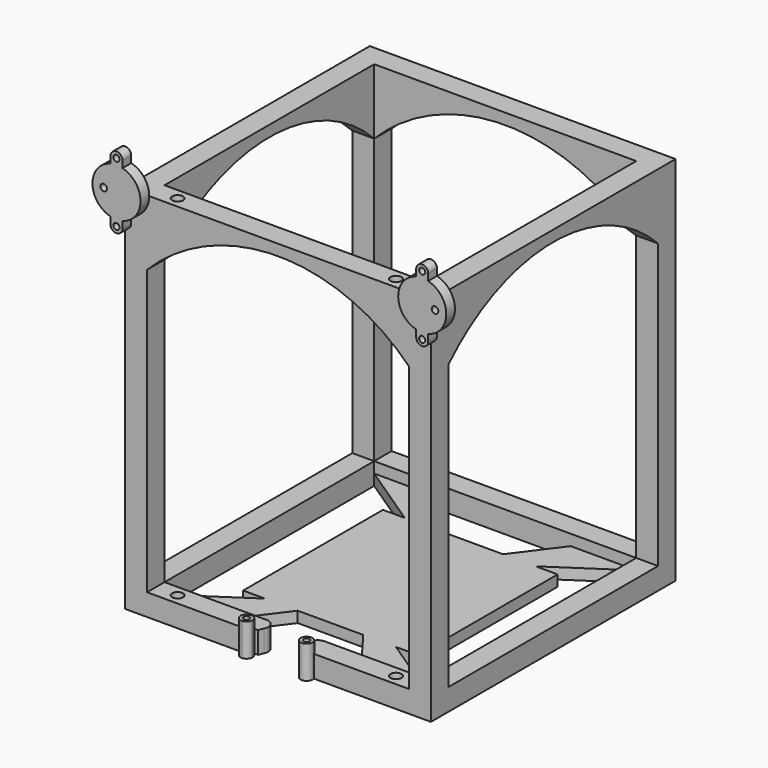
from build123d import *

# Parameters (mm, degrees)
F0_W      = 101.6
F0_H      = 101.6
F1_DEPTH  = 6.35
F2_W      = 12.7
F2_H      = 12.7
F3_DEPTH  = 88.9
F5_W      = 12.7
F5_H      = 12.7
F6_DEPTH  = 76.2
F9_W      = 38.1
F9_H      = 6.35
F8_W      = 19.05
F8_H      = 6.35
F14_W     = 12.7
F14_H     = 12.7
F15_DEPTH = 203.2
F17_DEPTH = 12.7
F20_DEPTH = 12.7
F22_R     = 3.175
F23_DEPTH = 209.55
F24_R     = 1.905
F24_R_2   = 1.778
F25_DEPTH = 19.05
F27_DEPTH = 25.4
F28_R     = 5.08
F29_R     = 1.778
F29_R_2   = 1.905
F30_DEPTH = 6.35


# Not quite as in the source:
# - a feature of the source that left no trace in its solid (it failed there, or was rolled back) is left out


with BuildPart() as f1:
    # F0 (on Top) → F1 (new body)
    with BuildSketch(Plane.XY):
        Rectangle(F0_W, F0_H)
    extrude(amount=-F1_DEPTH)



with BuildPart() as f3:
    # F2 (on Right) → F3 (new body, symmetric)
    with BuildSketch(Plane.YZ):
        with Locations((-82.55, 0)):
            Rectangle(F2_W, F2_H)
    extrude(amount=F3_DEPTH, both=True)


with BuildPart() as f4_1:
    # F4: instance of F3
    add(f3.part.mirror(Plane.XZ))


with BuildPart() as f3_1:
    add(f3.part)

    add(f4_1.part)  # F6 merges F4_1
    # F5 (on Front) → F6 (join, symmetric)
    with BuildSketch(Plane.XZ):
        with Locations((82.55, 0)):
            Rectangle(F5_W, F5_H)
    extrude(amount=F6_DEPTH, both=True)


with BuildPart() as f7_1:
    # F7: instance of F3
    add(f3_1.part.mirror(Plane.YZ))


with BuildPart() as f1_1:
    add(f1.part)

    add(f3_1.part)  # F10 merges F3

    add(f7_1.part)  # F10 merges F7_1
    # F9 (on face) → F10 section 0
    with BuildSketch(Plane(origin=(0, -76.2, 0), x_dir=(-1, 0, 0), z_dir=(0, 1, 0))):
        with Locations((57.15, -3.175)):
            Rectangle(F9_W, F9_H)
    # F8 (on face) → F10 section 1
    with BuildSketch(Plane.XZ.offset(50.8)):
        with Locations((-28.575, -3.175)):
            Rectangle(F8_W, F8_H)
    loft()


with BuildPart() as f11_1:
    # F11: instance of F1
    add(f1_1.part.mirror(Plane.YZ))


with BuildPart() as f12_1:
    # F12: instance of F11_1
    add(f11_1.part.mirror(Plane.XZ))


with BuildPart() as f12_2:
    # F12: instance of F1
    add(f1_1.part.mirror(Plane.XZ))


with BuildPart() as f1_2:
    add(f1_1.part)

    # F13: union F12_2, F11_1, F12_1
    add(f12_2.part)
    add(f11_1.part)
    add(f12_1.part)

    # F14 (on face) → F15 (join)
    with BuildSketch(Plane.XY.offset(6.35)):
        with Locations((-82.55, 82.55)):
            Rectangle(F14_W, F14_H)
        with Locations((82.55, 82.55)):
            Rectangle(F14_W, F14_H)
        with Locations((82.55, -82.55)):
            Rectangle(F14_W, F14_H)
        with Locations((-82.55, -82.55)):
            Rectangle(F14_W, F14_H)
    extrude(amount=F15_DEPTH)

    # F16 (on face) → F17 (join)
    with BuildSketch(Plane(origin=(-88.9, 0, 0), x_dir=(0, -1, 0), z_dir=(-1, 0, 0))):
        with BuildLine():
            ThreePointArc((-76.2, 171.45), (0, 203.2), (76.2, 171.45))
            Line((76.2, 171.45), (76.2, 209.55))
            Line((76.2, 209.55), (-76.2, 209.55))
            Line((-76.2, 209.55), (-76.2, 171.45))
        make_face()
    extrude(amount=-F17_DEPTH)

    # F18: F1 across plane


with BuildPart() as f1_3:
    add(f1_2.part)
    add(f1_2.part.mirror(Plane.YZ))

    # F19 (on face) → F20 (join)
    with BuildSketch(Plane(origin=(0, 88.9, 0), x_dir=(-1, 0, 0), z_dir=(0, 1, 0))):
        with BuildLine():
            ThreePointArc((-76.2, 171.45), (0, 203.2), (76.2, 171.45))
            Line((76.2, 171.45), (76.2, 209.55))
            Line((76.2, 209.55), (-76.2, 209.55))
            Line((-76.2, 209.55), (-76.2, 171.45))
        make_face()
    extrude(amount=-F20_DEPTH)

    # F21: F1 across plane


with BuildPart() as f1_4:
    add(f1_3.part)
    add(f1_3.part.mirror(Plane.XZ))

    # F22 (on face) → F23 (cut)
    with BuildSketch(Plane.XY.offset(209.55)):
        with Locations((-63.5, -82.55)):
            Circle(F22_R)
        with Locations((63.5, -82.55)):
            Circle(F22_R)
    extrude(amount=-F23_DEPTH, mode=Mode.SUBTRACT)

    # F24 (on face) → F25 (join)
    with BuildSketch(Plane(origin=(0, 0, -6.35), x_dir=(1, 0, 0), z_dir=(0, 0, -1))):
        with BuildLine():
            Line((17.45107, 93.48597), (13.5244245713, 93.48597))
            ThreePointArc((13.5244245713, 93.48597), (0, 103.95585), (-13.5244245713, 93.48597))
            Line((-13.5244245713, 93.48597), (-17.45107, 93.48597))
            ThreePointArc((-17.45107, 93.48597), (-20.95119, 89.98585), (-17.45107, 86.48573))
            Line((-17.45107, 86.48573), (-13.5244245713, 86.48573))
            ThreePointArc((-13.5244245713, 86.48573), (0, 76.01585), (13.5244245713, 86.48573))
            Line((13.5244245713, 86.48573), (17.45107, 86.48573))
            ThreePointArc((17.45107, 86.48573), (20.95119, 89.98585), (17.45107, 93.48597))
        make_face()
        with Locations((0, 82.55)):
            Circle(F24_R, mode=Mode.SUBTRACT)
        with Locations((-17.45107, 89.98585)):
            Circle(F24_R_2, mode=Mode.SUBTRACT)
        with Locations((17.45107, 89.98585)):
            Circle(F24_R_2, mode=Mode.SUBTRACT)
    extrude(amount=-F25_DEPTH)

    # F26 (on face) → F27 (cut)
    with BuildSketch(Plane.XY.offset(12.7)):
        with BuildLine():
            ThreePointArc((-17.45107, -86.48573), (-15.0942845585, -87.3981092098), (-13.9661895841, -89.6595855349))
            ThreePointArc((-13.9661895841, -89.6595855349), (-13.97, -89.98585), (-13.9661895841, -90.3121144651))
            ThreePointArc((-13.9661895841, -90.3121144651), (-15.0942845585, -92.5735907902), (-17.45107, -93.48597))
            Line((-17.45107, -93.48597), (-13.5244245713, -93.48597))
            ThreePointArc((-13.5244245713, -93.48597), (0, -103.95585), (13.5244245713, -93.48597))
            Line((13.5244245713, -93.48597), (17.45107, -93.48597))
            ThreePointArc((17.45107, -93.48597), (13.95095, -89.98585), (17.45107, -86.48573))
            Line((17.45107, -86.48573), (13.5244245713, -86.48573))
            ThreePointArc((13.5244245713, -86.48573), (0, -76.01585), (-13.5244245713, -86.48573))
            Line((-13.5244245713, -86.48573), (-17.45107, -86.48573))
        make_face()
    extrude(amount=-F27_DEPTH, mode=Mode.SUBTRACT)

    # F28
    f28_edges = [f1_4.edges().sort_by_distance(p)[0] for p in [
        (2.260805, -76.2, 0),
        (-2.260805, -76.2, 0),
    ]]
    fillet(f28_edges, radius=F28_R)

    # F29 (on face) → F30 (join)
    with BuildSketch(Plane.XZ.offset(88.9)):
        with BuildLine():
            Line((-85.39988, 192.09893), (-85.39988, 196.0255754287))
            ThreePointArc((-85.39988, 196.0255754287), (-74.93, 209.55), (-85.39988, 223.0744245713))
            Line((-85.39988, 223.0744245713), (-85.39988, 227.00107))
            ThreePointArc((-85.39988, 227.00107), (-88.9, 230.50119), (-92.40012, 227.00107))
            Line((-92.40012, 227.00107), (-92.40012, 223.0744245713))
            ThreePointArc((-92.40012, 223.0744245713), (-102.87, 209.55), (-92.40012, 196.0255754287))
            Line((-92.40012, 196.0255754287), (-92.40012, 192.09893))
            ThreePointArc((-92.40012, 192.09893), (-88.9, 188.59881), (-85.39988, 192.09893))
        make_face()
        with Locations((-88.9, 192.09893)):
            Circle(F29_R, mode=Mode.SUBTRACT)
        with Locations((-96.33585, 209.55)):
            Circle(F29_R_2, mode=Mode.SUBTRACT)
        with Locations((-88.9, 227.00107)):
            Circle(F29_R, mode=Mode.SUBTRACT)
        with BuildLine():
            Line((85.39988, 227.00107), (85.39988, 223.0744245713))
            ThreePointArc((85.39988, 223.0744245713), (74.93, 209.55), (85.39988, 196.0255754287))
            Line((85.39988, 196.0255754287), (85.39988, 192.09893))
            ThreePointArc((85.39988, 192.09893), (88.9, 188.59881), (92.40012, 192.09893))
            Line((92.40012, 192.09893), (92.40012, 196.0255754287))
            ThreePointArc((92.40012, 196.0255754287), (102.87, 209.55), (92.40012, 223.0744245713))
            Line((92.40012, 223.0744245713), (92.40012, 227.00107))
            ThreePointArc((92.40012, 227.00107), (88.9, 230.50119), (85.39988, 227.00107))
        make_face()
        with Locations((88.9, 192.09893)):
            Circle(F29_R, mode=Mode.SUBTRACT)
        with Locations((96.33585, 209.55)):
            Circle(F29_R_2, mode=Mode.SUBTRACT)
        with Locations((88.9, 227.00107)):
            Circle(F29_R, mode=Mode.SUBTRACT)
    extrude(amount=F30_DEPTH)


solid = f1_4.part
